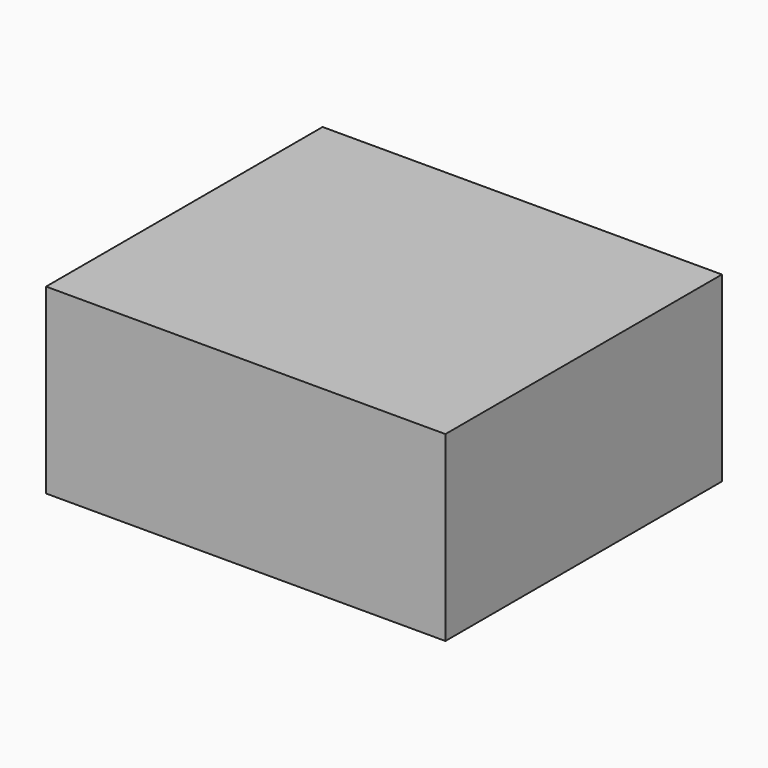
from build123d import *

# Parameters (mm, degrees)
F1_E0_TOP_W = 113.5742664337
F1_E0_TOP_H = 98.298
F2_DEPTH    = 51.816


with BuildPart() as f2:
    # F1_E0_top (on explicit) → F2 (new body)
    with BuildSketch(Plane(origin=(-55.3310513496, 0, -66.8158754706), x_dir=(1, 0, 0), z_dir=(0, 0, -1))):
        with Locations((56.7871332169, 49.149)):
            Rectangle(F1_E0_TOP_W, F1_E0_TOP_H)
    extrude(amount=-F2_DEPTH)


solid = f2.part
